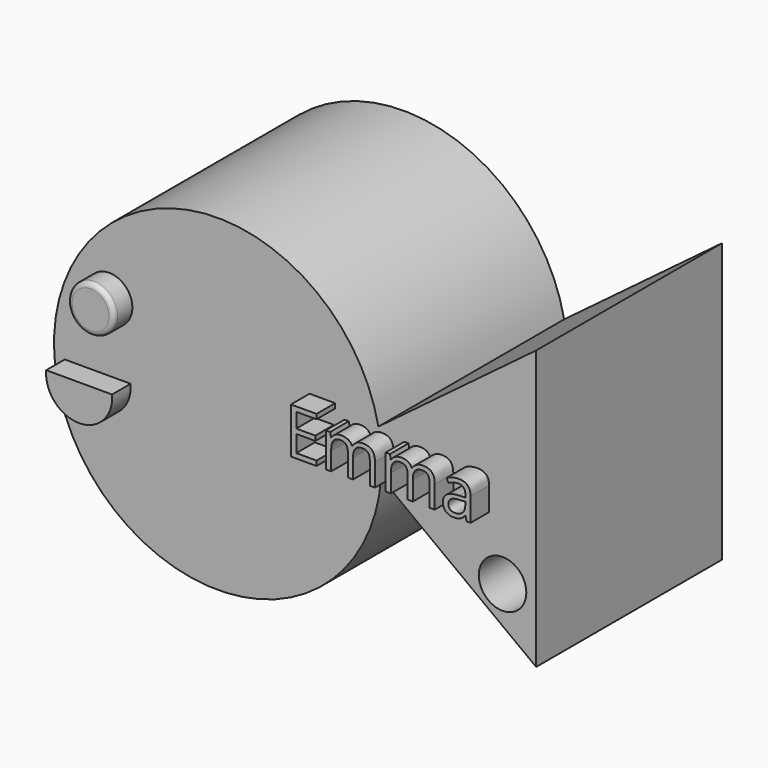
from build123d import *

# Parameters (mm, degrees)
F1_DEPTH     = 25.4
F2_R         = 2.5307293265
F3_DEPTH     = 2.54
F5_DEPTH     = 2.54
F6_TEXT_SIZE = 7.0298038837
F7_DEPTH     = 2.54
F8_R         = 2.59724156
F9_DEPTH     = 25.4
F10_R        = 0.508


# Not quite as in the source:
# - Text() gives the source's letters only with a copy of the font that has no kerning and outlines rounded to 1/6400 em; it was checked with that copy


with BuildPart() as f1:
    # F0 (on Front) → F1 (new body)
    with BuildSketch(Plane.XZ):
        with BuildLine():
            ThreePointArc((32.0791687439, 18.7561053322), (32.1143127978, 19.4032129836), (32.1260325929, 20.0511682779))
            ThreePointArc((32.1260325929, 20.0511682779), (32.0382499151, 21.8226141843), (31.7757620143, 23.5767026941))
            Line((31.7757620143, 23.5767026941), (28.7137338045, 21.2801815367))
            Line((28.7137338045, 21.2801815367), (32.0791687439, 18.7561053322))
        make_face()
        with BuildLine():
            ThreePointArc((31.7757620143, 23.5767026941), (32.0382499151, 21.8226141843), (32.1260325929, 20.0511682779))
            ThreePointArc((32.1260325929, 20.0511682779), (32.1143127978, 19.4032129836), (32.0791687439, 18.7561053322))
            Line((32.0791687439, 18.7561053322), (49.0337338045, 6.0401815367))
            Line((49.0337338045, 6.0401815367), (49.0337338045, 36.5201815367))
            Line((49.0337338045, 36.5201815367), (31.7757620143, 23.5767026941))
        make_face()
        with BuildLine():
            Line((28.7137338045, 21.2801815367), (31.7757620143, 23.5767026941))
            ThreePointArc((31.7757620143, 23.5767026941), (-3.6739718072, 18.925661878), (32.0791687439, 18.7561053322))
            Line((32.0791687439, 18.7561053322), (28.7137338045, 21.2801815367))
        make_face()
    extrude(amount=-F1_DEPTH)

    # F2 (on Front) → F3 (join)
    with BuildSketch(Plane.XZ):
        with Locations((2.3360580672, 26.2806583196)):
            Circle(F2_R)
    extrude(amount=F3_DEPTH)

    # F4 (on Front) → F5 (join)
    with BuildSketch(Plane.XZ):
        with BuildLine():
            Line((4.6721161343, 18.883138895), (-2.5307303295, 18.883138895))
            ThreePointArc((-2.5307303295, 18.883138895), (1.0706929024, 14.9556842568), (4.6721161343, 18.883138895))
        make_face()
    extrude(amount=F5_DEPTH)

    # F6 (on Front) → F7 (join)
    with BuildSketch(Plane.XZ):
        with Locations((23.5552564263, 19.2724820226)):
            Text('Emma', F6_TEXT_SIZE, font='Open Sans', text_align=(TextAlign.LEFT, TextAlign.BOTTOM))
    extrude(amount=F7_DEPTH)

    # F8 (on Front) → F9 (cut)
    with BuildSketch(Plane.XZ):
        with Locations((45.3584678471, 12.8483213484)):
            Circle(F8_R)
    extrude(amount=-F9_DEPTH, mode=Mode.SUBTRACT)

    # F10
    f10_edges = [f1.edges().sort_by_distance(p)[0] for p in [
        (-0.194671, -2.54, 26.280658),
    ]]
    fillet(f10_edges, radius=F10_R)


solid = f1.part
